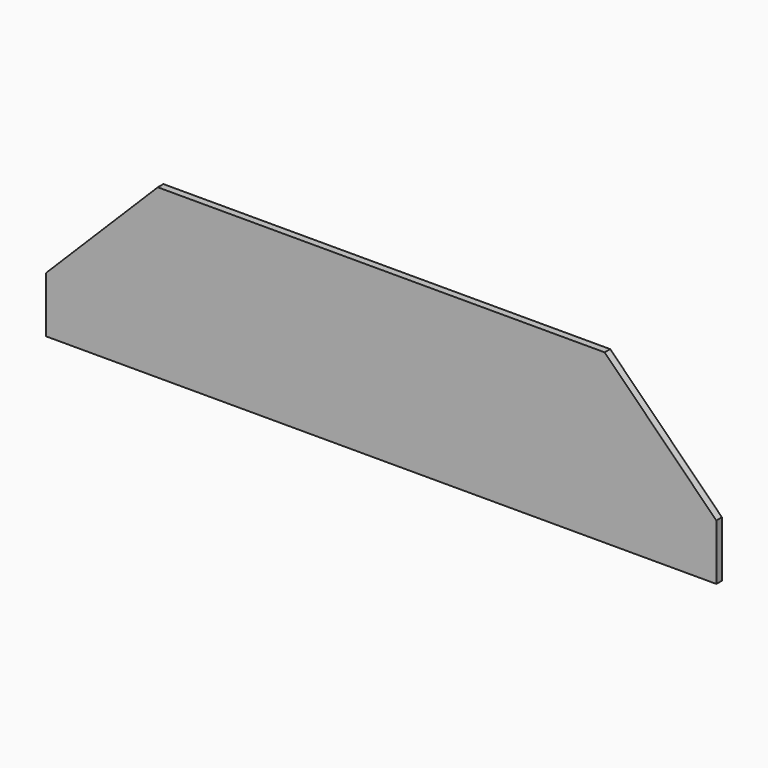
from build123d import *

# Parameters (mm, degrees)
F1_DEPTH = 3.175


# Not quite as in the source:
# - a feature names something its author has since deleted; it is built from what else it names


with BuildPart() as f1:
    # F0 (on Front) → F1 (new body)
    with BuildSketch(Plane.XZ):
        Polygon((304.8, -25.4), (304.8, 0), (254, 50.8), (50.8, 50.8), (0, 0), (0, -25.4), align=None)
    extrude(amount=F1_DEPTH)


solid = f1.part
